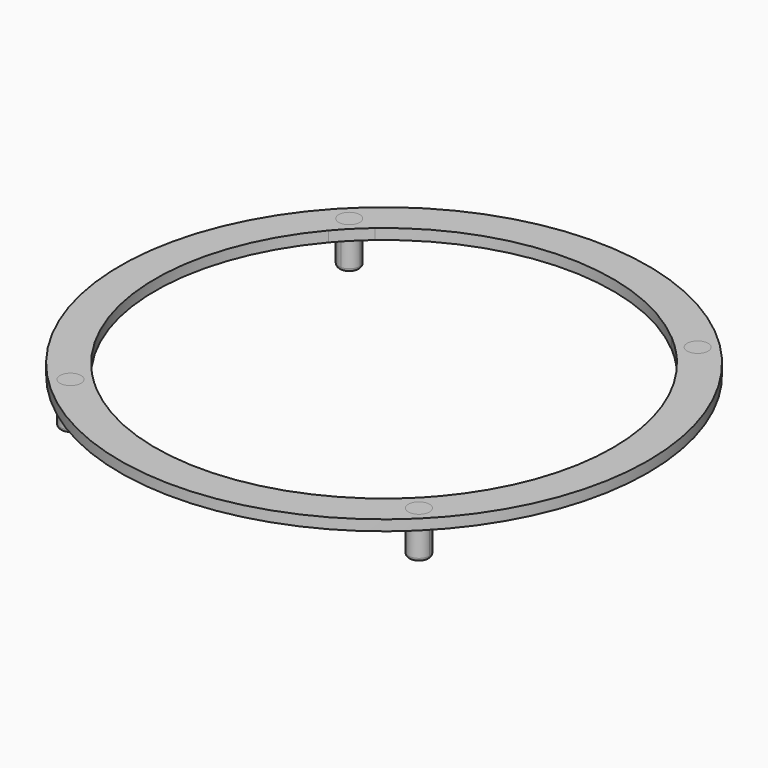
from build123d import *

# Parameters (mm, degrees)
F2_DEPTH = 6
F1_R     = 37.5
F4_DEPTH = 1.5


# Not quite as in the source:
# - a fillet or chamfer that OpenCascade refuses, or shapes differently, is made with other operations: its cross-section is extruded or revolved along the edge and cut away or added


with BuildPart() as f2:
    # F1 (on offset) → F2 (new body)
    with BuildSketch(Plane.XY.offset(-1)):
        with BuildLine():
            Line((-24.75, 24.75), (-23.25, 24.75))
            ThreePointArc((-23.25, 24.75), (-25.8106601718, 25.8106601718), (-24.75, 23.25))
            Line((-24.75, 23.25), (-24.75, 24.75))
        make_face()
        with BuildLine():
            ThreePointArc((-24.75, 23.25), (-23.6893398282, 23.6893398282), (-23.25, 24.75))
            Line((-23.25, 24.75), (-24.75, 24.75))
            Line((-24.75, 24.75), (-24.75, 23.25))
        make_face()
    extrude(amount=-F2_DEPTH)

    # F3: fillet of radius 0.5 on 1 edges, made by hand

    # F3_s1 → F3_t2 (revolve, cut)
    with BuildSketch(Plane.YZ.offset(-24.75)):
        with BuildLine():
            ThreePointArc((23.25, -6.5), (23.3964466094, -6.8535533906), (23.75, -7))
            Line((23.75, -7), (23.25, -7))
            Line((23.25, -7), (23.25, -6.5))
        make_face()
    revolve(axis=Axis((-24.75, 24.75, -7), (0, 0, 1)), mode=Mode.SUBTRACT)


with BuildPart() as f2b:
    # F1 (on offset) → F2, piece 2 (new body)
    with BuildSketch(Plane.XY.offset(-1)):
        with BuildLine():
            ThreePointArc((23.25, 24.75), (23.6893398282, 23.6893398282), (24.75, 23.25))
            Line((24.75, 23.25), (24.75, 24.75))
            Line((24.75, 24.75), (23.25, 24.75))
        make_face()
        with BuildLine():
            Line((24.75, 24.75), (24.75, 23.25))
            ThreePointArc((24.75, 23.25), (25.8106601718, 23.6893398282), (26.25, 24.75))
            ThreePointArc((26.25, 24.75), (24.75, 26.25), (23.25, 24.75))
            Line((23.25, 24.75), (24.75, 24.75))
        make_face()
    extrude(amount=-F2_DEPTH)

    # F3#2: fillet of radius 0.5 on 1 edges, made by hand

    # F3_2_s1 → F3_2_t2 (revolve, cut)
    with BuildSketch(Plane.YZ.offset(24.75)):
        with BuildLine():
            ThreePointArc((23.25, -6.5), (23.3964466094, -6.8535533906), (23.75, -7))
            Line((23.75, -7), (23.25, -7))
            Line((23.25, -7), (23.25, -6.5))
        make_face()
    revolve(axis=Axis((24.75, 24.75, -7), (0, 0, 1)), mode=Mode.SUBTRACT)


with BuildPart() as f2c:
    # F1 (on offset) → F2, piece 3 (new body)
    with BuildSketch(Plane.XY.offset(-1)):
        with BuildLine():
            ThreePointArc((26.25, -24.75), (25.8106601718, -23.6893398282), (24.75, -23.25))
            Line((24.75, -23.25), (24.75, -24.75))
            Line((24.75, -24.75), (23.25, -24.75))
            ThreePointArc((23.25, -24.75), (24.75, -26.25), (26.25, -24.75))
        make_face()
        with BuildLine():
            Line((24.75, -24.75), (24.75, -23.25))
            ThreePointArc((24.75, -23.25), (23.6893398282, -23.6893398282), (23.25, -24.75))
            Line((23.25, -24.75), (24.75, -24.75))
        make_face()
    extrude(amount=-F2_DEPTH)

    # F3#3: fillet of radius 0.5 on 1 edges, made by hand

    # F3_3_s1 → F3_3_t2 (revolve, cut)
    with BuildSketch(Plane.XZ.offset(24.75)):
        with BuildLine():
            ThreePointArc((26.25, -6.5), (26.1035533906, -6.8535533906), (25.75, -7))
            Line((25.75, -7), (26.25, -7))
            Line((26.25, -7), (26.25, -6.5))
        make_face()
    revolve(axis=Axis((24.75, -24.75, -7), (0, 0, 1)), mode=Mode.SUBTRACT)


with BuildPart() as f2d:
    # F1 (on offset) → F2, piece 4 (new body)
    with BuildSketch(Plane.XY.offset(-1)):
        with BuildLine():
            Line((-24.75, -24.75), (-23.25, -24.75))
            ThreePointArc((-23.25, -24.75), (-23.6893398282, -23.6893398282), (-24.75, -23.25))
            Line((-24.75, -23.25), (-24.75, -24.75))
        make_face()
        with BuildLine():
            ThreePointArc((-24.75, -23.25), (-25.8106601718, -25.8106601718), (-23.25, -24.75))
            Line((-23.25, -24.75), (-24.75, -24.75))
            Line((-24.75, -24.75), (-24.75, -23.25))
        make_face()
    extrude(amount=-F2_DEPTH)

    # F3#4: fillet of radius 0.5 on 1 edges, made by hand

    # F3_4_s1 → F3_4_t2 (revolve, cut)
    with BuildSketch(Plane.YZ.offset(-24.75)):
        with BuildLine():
            ThreePointArc((-23.25, -6.5), (-23.3964466094, -6.8535533906), (-23.75, -7))
            Line((-23.75, -7), (-23.25, -7))
            Line((-23.25, -7), (-23.25, -6.5))
        make_face()
    revolve(axis=Axis((-24.75, -24.75, -7), (0, 0, 1)), mode=Mode.SUBTRACT)


with BuildPart() as f4:
    # F1 (on offset) → F4 (new body)
    with BuildSketch(Plane.XY.offset(-1)):
        Circle(F1_R)
        with BuildLine():
            ThreePointArc((24.75, 21.0638909036), (30.501024573, 11.2221878437), (32.5, 0))
            ThreePointArc((32.5, 0), (30.501024573, -11.2221878437), (24.75, -21.0638909036))
            Line((24.75, -21.0638909036), (24.75, -23.25))
            ThreePointArc((24.75, -23.25), (25.8106601718, -23.6893398282), (26.25, -24.75))
            ThreePointArc((26.25, -24.75), (24.75, -26.25), (23.25, -24.75))
            Line((23.25, -24.75), (21.0638909036, -24.75))
            ThreePointArc((21.0638909036, -24.75), (0, -32.5), (-21.0638909036, -24.75))
            Line((-21.0638909036, -24.75), (-23.25, -24.75))
            ThreePointArc((-23.25, -24.75), (-25.8106601718, -25.8106601718), (-24.75, -23.25))
            Line((-24.75, -23.25), (-24.75, -21.0638909036))
            ThreePointArc((-24.75, -21.0638909036), (-32.5, 0), (-24.75, 21.0638909036))
            Line((-24.75, 21.0638909036), (-24.75, 23.25))
            ThreePointArc((-24.75, 23.25), (-25.8106601718, 25.8106601718), (-23.25, 24.75))
            Line((-23.25, 24.75), (-21.0638909036, 24.75))
            ThreePointArc((-21.0638909036, 24.75), (0, 32.5), (21.0638909036, 24.75))
            Line((21.0638909036, 24.75), (23.25, 24.75))
            ThreePointArc((23.25, 24.75), (24.75, 26.25), (26.25, 24.75))
            ThreePointArc((26.25, 24.75), (25.8106601718, 23.6893398282), (24.75, 23.25))
            Line((24.75, 23.25), (24.75, 21.0638909036))
        make_face(mode=Mode.SUBTRACT)
        with BuildLine():
            Line((-23.25, -24.75), (-21.0638909036, -24.75))
            ThreePointArc((-21.0638909036, -24.75), (-22.9809703886, -22.9809703886), (-24.75, -21.0638909036))
            Line((-24.75, -21.0638909036), (-24.75, -23.25))
            ThreePointArc((-24.75, -23.25), (-23.6893398282, -23.6893398282), (-23.25, -24.75))
        make_face()
        with BuildLine():
            ThreePointArc((-24.75, 21.0638909036), (-22.9809703886, 22.9809703886), (-21.0638909036, 24.75))
            Line((-21.0638909036, 24.75), (-23.25, 24.75))
            ThreePointArc((-23.25, 24.75), (-23.6893398282, 23.6893398282), (-24.75, 23.25))
            Line((-24.75, 23.25), (-24.75, 21.0638909036))
        make_face()
        with BuildLine():
            ThreePointArc((21.0638909036, 24.75), (22.9809703886, 22.9809703886), (24.75, 21.0638909036))
            Line((24.75, 21.0638909036), (24.75, 23.25))
            ThreePointArc((24.75, 23.25), (23.6893398282, 23.6893398282), (23.25, 24.75))
            Line((23.25, 24.75), (21.0638909036, 24.75))
        make_face()
        with BuildLine():
            Line((24.75, -23.25), (24.75, -21.0638909036))
            ThreePointArc((24.75, -21.0638909036), (22.9809703886, -22.9809703886), (21.0638909036, -24.75))
            Line((21.0638909036, -24.75), (23.25, -24.75))
            ThreePointArc((23.25, -24.75), (23.6893398282, -23.6893398282), (24.75, -23.25))
        make_face()
    extrude(amount=-F4_DEPTH)


solid = Compound([f2.part, f2b.part, f2c.part, f2d.part, f4.part])
